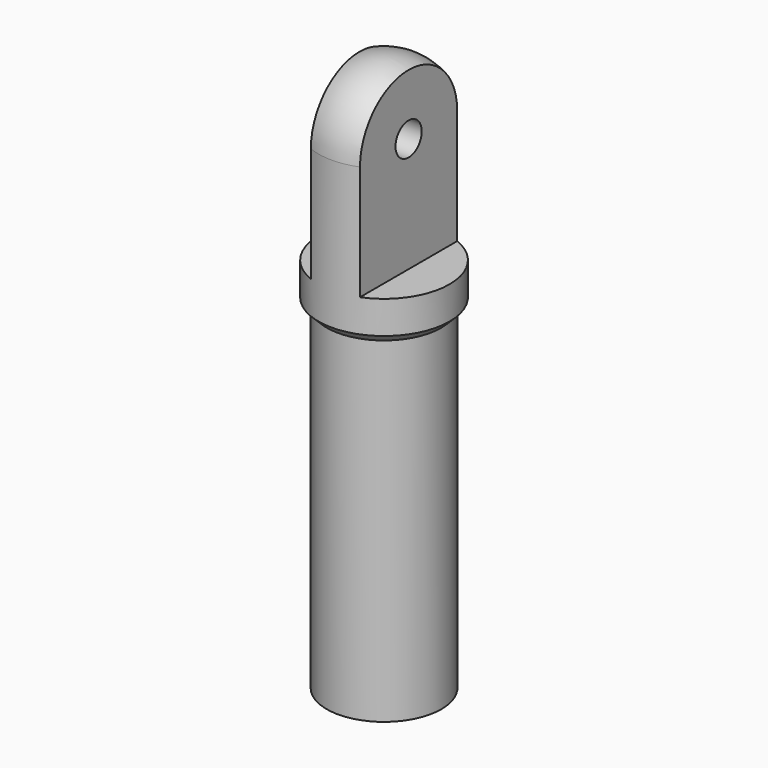
from build123d import *

# Parameters (mm, degrees)
F2_W     = 80.6665748954
F2_H     = 63.3093791263
F3_DEPTH = 100
F4_R     = 1
F5_DEPTH = 5.501


# Not quite as in the source:
# - a pattern or mirror of a feature is missing from the dataset's text; its kind, count and spacing are read off the source's solid


with BuildPart() as f1:
    # F0 (on Front) → F1 (revolve)
    with BuildSketch(Plane.XZ):
        with BuildLine():
            Line((2.05, -1), (2.05, -18))
            Line((2.05, -18), (3.5, -18))
            Line((3.5, -18), (3.5, 2.5))
            Line((3.5, 2.5), (4, 3))
            Line((4, 3), (4, 12))
            ThreePointArc((4, 12), (2.8284271247, 14.8284271247), (0, 16))
            Line((0, 16), (0, 12))
            Line((0, 12), (0, 0))
            Line((0, 0), (1.05, 0))
            ThreePointArc((1.05, 0), (1.7571067812, -0.2928932188), (2.05, -1))
        make_face()
    revolve(axis=Axis((0, 0, 14), (0, 0, -1)))

    # F2 (on Front) → F3 (cut, symmetric)
    with BuildSketch(Plane.XZ):
        with Locations((-41.8332874477, 36.6546895631)):
            Rectangle(F2_W, F2_H)
    f3 = extrude(amount=F3_DEPTH, both=True, mode=Mode.SUBTRACT)

    # F3_copies: F3 across plane
    add(f3.mirror(Plane(origin=(0, 0, 0), x_dir=(0, 0, 1), z_dir=(1, 0, 0))), mode=Mode.SUBTRACT)

    # F4 (on face) → F5 (cut, through all)
    with BuildSketch(Plane(origin=(-1.5, 0, 0), x_dir=(0, -1, 0), z_dir=(-1, 0, 0))):
        with Locations((0, 12)):
            Circle(F4_R)
    extrude(amount=-F5_DEPTH, mode=Mode.SUBTRACT)


solid = f1.part
